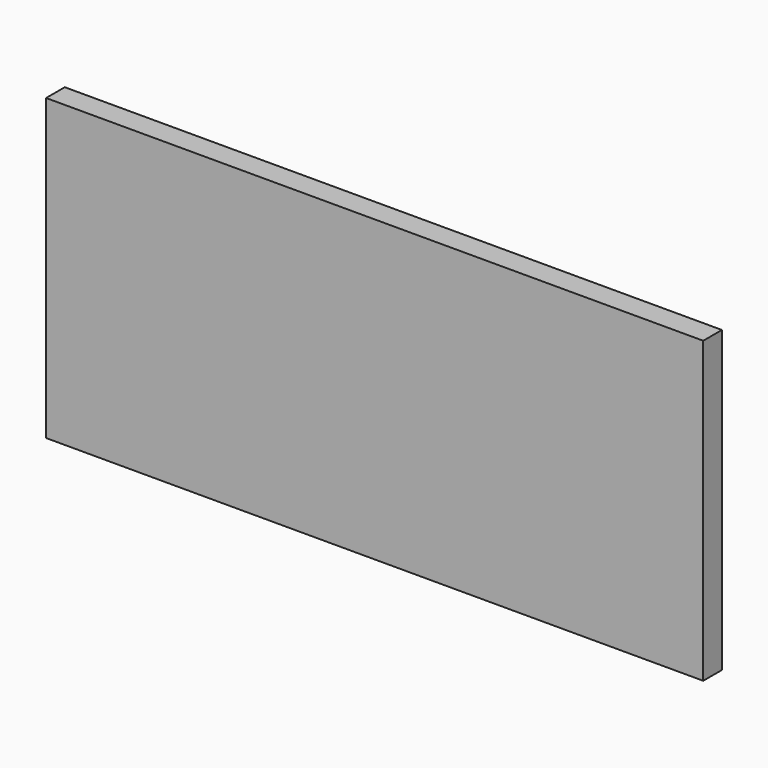
from build123d import *

# Parameters (mm, degrees)
F0_W     = 45
F0_H     = 20.5
F1_DEPTH = 1.6


# Not quite as in the source:
# - the program builds the solid bodies; features that only make, move or delete a surface that nothing else refers to are left out


with BuildPart() as f1:
    # F0 (on Front) → F1 (new body)
    with BuildSketch(Plane.XZ):
        Rectangle(F0_W, F0_H)
    extrude(amount=F1_DEPTH)


solid = f1.part
